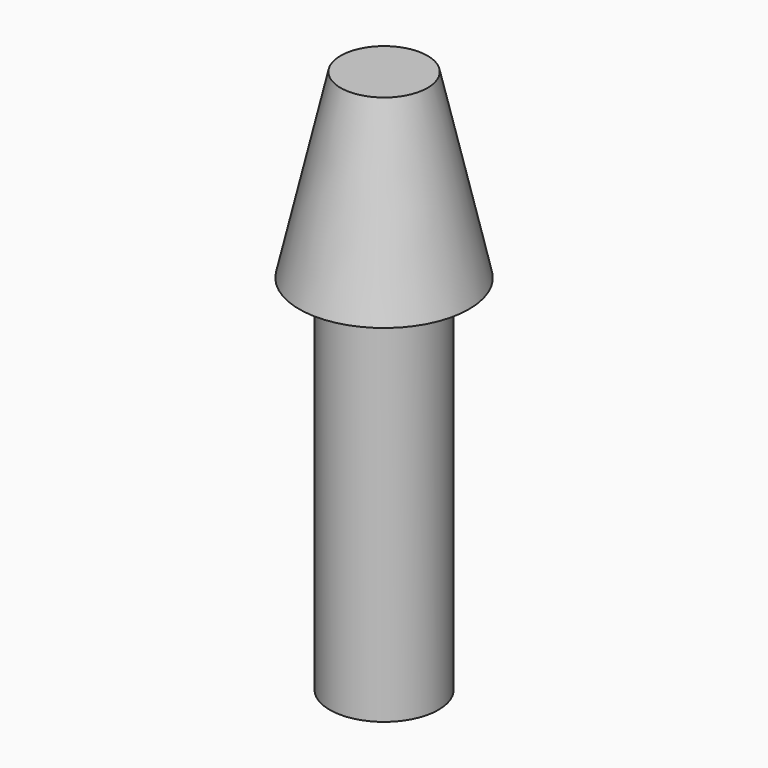
from build123d import *

# Parameters (mm, degrees)
F0_R     = 14
F1_DEPTH = 25
F3_R     = 7.5
F4_DEPTH = 50


# Not quite as in the source:
# - a fillet or chamfer that OpenCascade refuses, or shapes differently, is made with other operations: its cross-section is extruded or revolved along the edge and cut away or added


with BuildPart() as f1:
    # F0 (on Top) → F1 (new body)
    with BuildSketch(Plane.XY):
        Circle(F0_R)
    extrude(amount=F1_DEPTH)

    # F2: chamfer of 8 x 35 on 1 edges, made by hand

    # F2_s1 → F2_t2 (revolve, cut)
    with BuildSketch(Plane.XZ):
        Polygon((14, -10), (6, 25), (14, 25), align=None)
    revolve(axis=Axis((0, 0, 25), (0, 0, 1)), mode=Mode.SUBTRACT)

    # F3 (on face) → F4 (join)
    with BuildSketch(Plane(origin=(0, 0, 0), x_dir=(1, 0, 0), z_dir=(0, 0, -1))):
        Circle(F3_R)
    extrude(amount=F4_DEPTH)


solid = f1.part
